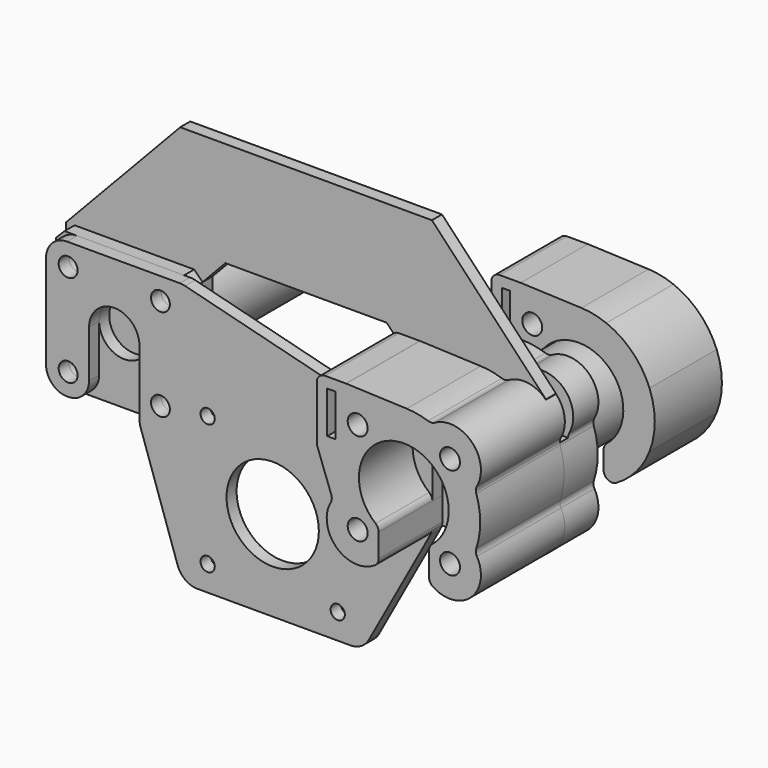
from build123d import *

# Parameters (mm, degrees)
F0_R           = 1.7
F0_R_2         = 11
F0_R_3         = 2.25
F1_DEPTH       = 3
F2_R           = 5
F3_W           = 32.5
F3_H           = 32.5
F3_R           = 2.25
F3_R_2         = 6
F4_DEPTH       = 3
F5_R           = 10.5
F5_R_2         = 6
F6_DEPTH       = 50
F7_SIZE        = 2
F10_R          = 2.375
F10_W          = 2
F10_H          = 10
F11_DEPTH      = 10
F13_R          = 2.375
F13_W          = 2
F13_H          = 10
F14_DEPTH      = 20
F12_W          = 2.5
F12_H          = 12.5
F15_DEPTH      = 36.626
F17_DEPTH      = 3
F18_F1_R       = 2
F18_F2_R       = 2
F18_2_T1_DEPTH = 25.630870957
F18_2_T3_DEPTH = 25.0205555548
F18_2_T5_DEPTH = 27.4736016845
F18_2_T7_DEPTH = 21.7710498822
F18_2_T9_DEPTH = 30
F19_R          = 2.25
F20_DEPTH      = 3
F21_R          = 1.99999
F21_R_2        = 2
F22_R          = 2.375
F23_DEPTH      = 3
F24_R          = 3.5
F26_R          = 2.375
F27_DEPTH      = 25


# Not quite as in the source:
# - a fillet or chamfer that OpenCascade refuses, or shapes differently, is made with other operations: its cross-section is extruded or revolved along the edge and cut away or added
# - a fillet or chamfer is up to 0.001 mm smaller than in the source, because OpenCascade refuses the exact size
# - an extrude whose draft closes it to a point is written as a loft to that point


with BuildPart() as f1:
    # F0 (on Front) → F1 (new body)
    with BuildSketch(Plane.XZ):
        with BuildLine():
            Line((-24.65, 16.25), (-57.15, 16.25))
            Line((-57.15, 16.25), (-57.15, -16.25))
            Line((-57.15, -16.25), (-46.9, -16.25))
            Line((-46.9, -16.25), (-46.9, 0))
            ThreePointArc((-46.9, 0), (-40.9, 6), (-34.9, 0))
            Line((-34.9, 0), (-34.9, -16.25))
            Line((-34.9, -16.25), (-24.65, -46.5))
            Line((-24.65, -46.5), (18.35, -46.5))
            Line((18.35, -46.5), (34.9, -16.25))
            Line((34.9, -16.25), (34.9, 0))
            ThreePointArc((34.9, 0), (40.9, 6), (46.9, 0))
            Line((46.9, 0), (46.9, -16.25))
            Line((46.9, -16.25), (57.15, -16.25))
            Line((57.15, -16.25), (57.15, 16.25))
            Line((57.15, 16.25), (24.65, 16.25))
            Line((24.65, 16.25), (24.65, 6.25))
            Line((24.65, 6.25), (14.65, 6.25))
            Line((14.65, 6.25), (-24.65, 16.25))
        make_face()
        with Locations((-18.65, -40.5)):
            Circle(F0_R, mode=Mode.SUBTRACT)
        with Locations((-3.15, -25)):
            Circle(F0_R_2, mode=Mode.SUBTRACT)
        with Locations((12.35, -40.5)):
            Circle(F0_R, mode=Mode.SUBTRACT)
        with Locations((-51.9, -11)):
            Circle(F0_R_3, mode=Mode.SUBTRACT)
        with Locations((-29.9, -11)):
            Circle(F0_R_3, mode=Mode.SUBTRACT)
        with Locations((-18.65, -9.5)):
            Circle(F0_R, mode=Mode.SUBTRACT)
        with Locations((-51.9, 11)):
            Circle(F0_R_3, mode=Mode.SUBTRACT)
        with Locations((-29.9, 11)):
            Circle(F0_R_3, mode=Mode.SUBTRACT)
        with Locations((12.35, -9.5)):
            Circle(F0_R, mode=Mode.SUBTRACT)
        with Locations((29.9, -11)):
            Circle(F0_R_3, mode=Mode.SUBTRACT)
        with Locations((51.9, -11)):
            Circle(F0_R_3, mode=Mode.SUBTRACT)
        with Locations((29.9, 11)):
            Circle(F0_R_3, mode=Mode.SUBTRACT)
        with Locations((51.9, 11)):
            Circle(F0_R_3, mode=Mode.SUBTRACT)
    extrude(amount=F1_DEPTH)

    # F2
    f2_edges = [f1.edges().sort_by_distance(p)[0] for p in [
        (-57.15, -1.5, -16.25),
        (-57.15, -1.5, 16.25),
        (-46.9, -1.5, -16.25),
        (-34.9, -1.5, -16.25),
        (-24.65, -1.5, -46.5),
        (18.35, -1.5, -46.5),
        (34.9, -1.5, -16.25),
        (46.9, -1.5, -16.25),
        (57.15, -1.5, -16.25),
        (57.15, -1.5, 16.25),
        (24.65, -1.5, 16.25),
        (14.65, -1.5, 6.25),
        (-24.65, -1.5, 16.25),
    ]]
    fillet(f2_edges, radius=F2_R)


with BuildPart() as f4:
    # F3 (on face) → F4 (new body)
    with BuildSketch(Plane(origin=(0, 0, 0), x_dir=(-1, 0, 0), z_dir=(0, 1, 0))):
        with Locations((-40.9, 0)):
            Rectangle(F3_W, F3_H)
        with Locations((-51.9, -11)):
            Circle(F3_R, mode=Mode.SUBTRACT)
        with Locations((-29.9, -11)):
            Circle(F3_R, mode=Mode.SUBTRACT)
        with Locations((-51.9, 11)):
            Circle(F3_R, mode=Mode.SUBTRACT)
        with Locations((-40.9, 0)):
            Circle(F3_R_2, mode=Mode.SUBTRACT)
        with Locations((-29.9, 11)):
            Circle(F3_R, mode=Mode.SUBTRACT)
    extrude(amount=F4_DEPTH)

    # F5 (on face) → F6 (join)
    with BuildSketch(Plane(origin=(0, 3, 0), x_dir=(-1, 0, 0), z_dir=(0, 1, 0))):
        with Locations((-40.9, 0)):
            Circle(F5_R)
        with Locations((-40.9, 0)):
            Circle(F5_R_2, mode=Mode.SUBTRACT)
    extrude(amount=F6_DEPTH)

    # F7
    f7_edges = [f4.edges().sort_by_distance(p)[0] for p in [
        (57.15, 1.5, 16.25),
        (24.65, 1.5, 16.25),
        (24.65, 1.5, -16.25),
        (57.15, 1.5, -16.25),
    ]]
    chamfer(f7_edges, length=F7_SIZE)


with BuildPart() as f8_1:
    # F8: instance of F4
    add(f4.part.mirror(Plane.YZ))


with BuildPart() as f11:
    # F10 (on offset) → F11 (new body)
    with BuildSketch(Plane(origin=(0, 6, 0), x_dir=(-1, 0, 0), z_dir=(0, 1, 0))):
        with BuildLine():
            ThreePointArc((-46.9, -8.8594582227), (-40.9, 10.7), (-34.9, -8.8594582227))
            Line((-34.9, -8.8594582227), (-34.9, -16.4213121106))
            ThreePointArc((-34.9, -16.4213121106), (-24.9853159914, -16.4987731446), (-23.9535532643, -6.6376157643))
            ThreePointArc((-23.9535532643, -6.6376157643), (-23.8791795551, -6.4445070705), (-23.8070062826, -6.2505652365))
            Line((-23.8070062826, -6.2505652365), (-20.15, 3.75))
            Line((-20.15, 3.75), (-20.15, 18.75))
            Line((-20.15, 18.75), (-27.15, 18.75))
            Line((-27.15, 18.75), (-41.609153009, 18.1861788733))
            ThreePointArc((-41.609153009, 18.1861788733), (-44.625317006, 17.8146572576), (-47.5376157643, 16.9464467357))
            ThreePointArc((-47.5376157643, 16.9464467357), (-57.1149125113, 16.2149125113), (-57.8464467357, 6.6376157643))
            ThreePointArc((-57.8464467357, 6.6376157643), (-59.1, 0), (-57.8464467357, -6.6376157643))
            ThreePointArc((-57.8464467357, -6.6376157643), (-56.8146840086, -16.4987731446), (-46.9, -16.4213121106))
            Line((-46.9, -16.4213121106), (-46.9, -8.8594582227))
        make_face()
        with Locations((-51.9, -11)):
            Circle(F10_R, mode=Mode.SUBTRACT)
        with Locations((-29.9, -11)):
            Circle(F10_R, mode=Mode.SUBTRACT)
        with Locations((-51.9, 11)):
            Circle(F10_R, mode=Mode.SUBTRACT)
        with Locations((-29.9, 11)):
            Circle(F10_R, mode=Mode.SUBTRACT)
        with Locations((-23.65, 11.25)):
            Rectangle(F10_W, F10_H, mode=Mode.SUBTRACT)
    extrude(amount=F11_DEPTH)

    # F12 (on face) → F15 (cut, through all)
    with BuildSketch(Plane.YZ.offset(22.65)):
        with Locations((7.25, 12.5)):
            Rectangle(F12_W, F12_H)
    extrude(amount=F15_DEPTH, mode=Mode.SUBTRACT)

    # F16 (on face) → F17 (cut)
    with BuildSketch(Plane(origin=(0, 16, 0), x_dir=(-1, 0, 0), z_dir=(0, 1, 0))):
        Polygon((-47.9962572492, 9.9539952825), (-49.0422619668, 13.8577380332), (-52.9460047175, 14.9037427508), (-55.8037427508, 12.0460047175), (-54.7577380332, 8.1422619668), (-50.8539952825, 7.0962572492), align=None)
        Polygon((-50.8539952825, -7.0962572492), (-54.7577380332, -8.1422619668), (-55.8037427508, -12.0460047175), (-52.9460047175, -14.9037427508), (-49.0422619668, -13.8577380332), (-47.9962572492, -9.9539952825), align=None)
    extrude(amount=-F17_DEPTH, mode=Mode.SUBTRACT)

    # F18: fillet of radius 2 on 11 edges, made by hand

    # F18_f1
    f18_f1_edges = [f11.edges().sort_by_distance(p)[0] for p in [
        (47.5376157643, 12.25, 16.9464467357),
        (57.8464467357, 12.25, 6.6376157643),
        (57.8464467357, 11, -6.6376157643),
        (23.9535532643, 11, -6.6376157643),
    ]]
    fillet(f18_f1_edges, radius=F18_F1_R)

    # F18_f2
    f18_f2_edges = [f11.edges().sort_by_distance(p)[0] for p in [
        (46.9, 11, -16.4213121106),
        (46.9, 11, -8.8594582227),
        (20.15, 11, 3.75),
        (20.15, 11, 18.75),
        (27.15, 12.25, 18.75),
        (34.9, 11, -8.8594582227),
        (34.9, 11, -16.4213121106),
    ]]
    fillet(f18_f2_edges, radius=F18_F2_R)

    # F24 (on face) → F25 section 0
    with BuildSketch(Plane(origin=(0, 16, 0), x_dir=(-1, 0, 0), z_dir=(0, 1, 0)), mode=Mode.PRIVATE) as f25_s0:
        with Locations((-29.9, -11)):
            Circle(F24_R)
    loft([f25_s0.sketch, Vertex(29.9, 12.5, -11)], ruled=True, mode=Mode.SUBTRACT)


with BuildPart() as f14:
    # F13 (on face) → F14 (new body)
    with BuildSketch(Plane(origin=(0, 53, 0), x_dir=(-1, 0, 0), z_dir=(0, 1, 0))):
        with BuildLine():
            Line((-27.15, 18.75), (-41.609153009, 18.1861788733))
            ThreePointArc((-41.609153009, 18.1861788733), (-44.625317006, 17.8146572576), (-47.5376157643, 16.9464467357))
            ThreePointArc((-47.5376157643, 16.9464467357), (-53.7693434176, 12.8693434176), (-57.8464467357, 6.6376157643))
            ThreePointArc((-57.8464467357, 6.6376157643), (-59.1, 0), (-57.8464467357, -6.6376157643))
            ThreePointArc((-57.8464467357, -6.6376157643), (-53.7693434176, -12.8693434176), (-47.5376157643, -16.9464467357))
            ThreePointArc((-47.5376157643, -16.9464467357), (-47.2114499856, -16.6928133434), (-46.9, -16.4213121106))
            Line((-46.9, -16.4213121106), (-46.9, -8.8594582227))
            ThreePointArc((-46.9, -8.8594582227), (-40.9, 10.7), (-34.9, -8.8594582227))
            Line((-34.9, -8.8594582227), (-34.9, -16.4213121106))
            ThreePointArc((-34.9, -16.4213121106), (-34.5885500144, -16.6928133434), (-34.2623842357, -16.9464467357))
            ThreePointArc((-34.2623842357, -16.9464467357), (-28.0306565824, -12.8693434176), (-23.9535532643, -6.6376157643))
            ThreePointArc((-23.9535532643, -6.6376157643), (-23.8791795551, -6.4445070705), (-23.8070062826, -6.2505652365))
            Line((-23.8070062826, -6.2505652365), (-20.15, 3.75))
            Line((-20.15, 3.75), (-20.15, 18.75))
            Line((-20.15, 18.75), (-27.15, 18.75))
        make_face()
        with Locations((-29.9, 11)):
            Circle(F13_R, mode=Mode.SUBTRACT)
        with Locations((-23.65, 11.25)):
            Rectangle(F13_W, F13_H, mode=Mode.SUBTRACT)
    extrude(amount=-F14_DEPTH)

    # F18#2: fillet of radius 2 on 6 edges, made by hand

    # F18_2_s2 → F18_2_t1 (cut)
    with BuildSketch(Plane.XZ.offset(-55.8154354785)):
        with BuildLine():
            ThreePointArc((46.9, -15.4598906937), (47.1347014219, -16.3999550161), (47.7837209302, -17.1193849053))
            ThreePointArc((47.7837209302, -17.1193849053), (47.3285163868, -16.7872413613), (46.9, -16.4213121106))
            Line((46.9, -16.4213121106), (46.9, -15.4598906937))
        make_face()
    extrude(amount=F18_2_T1_DEPTH, mode=Mode.SUBTRACT)

    # F18_2_s4 → F18_2_t3 (cut)
    with BuildSketch(Plane.XZ.offset(-55.5102777774)):
        with BuildLine():
            ThreePointArc((47.6401574803, -8.3102513284), (47.0944966021, -9.0032452783), (46.9, -9.8635693337))
            Line((46.9, -9.8635693337), (46.9, -8.8594582227))
            ThreePointArc((46.9, -8.8594582227), (47.2759948407, -8.5928278111), (47.6401574803, -8.3102513284))
        make_face()
        with BuildLine():
            ThreePointArc((34.9, -9.8635693337), (34.7055033979, -9.0032452783), (34.1598425197, -8.3102513284))
            ThreePointArc((34.1598425197, -8.3102513284), (34.5240051593, -8.5928278111), (34.9, -8.8594582227))
            Line((34.9, -8.8594582227), (34.9, -9.8635693337))
        make_face()
    extrude(amount=F18_2_T3_DEPTH, mode=Mode.SUBTRACT)

    # F18_2_s6 → F18_2_t5 (cut)
    with BuildSketch(Plane.XZ.offset(-56.7368008423)):
        with BuildLine():
            ThreePointArc((35.3717736883, -15.9447262517), (34.2737734044, -16.5662065114), (33.0222118523, -16.4067197788))
            ThreePointArc((33.0222118523, -16.4067197788), (33.6372826037, -16.6881076225), (34.2623842357, -16.9464467357))
            ThreePointArc((34.2623842357, -16.9464467357), (34.8425222812, -16.4737645638), (35.3717736883, -15.9447262517))
        make_face()
    extrude(amount=F18_2_T5_DEPTH, mode=Mode.SUBTRACT)

    # F18_2_s8 → F18_2_t7 (cut)
    with BuildSketch(Plane.XZ.offset(-53.8855249411)):
        with BuildLine():
            ThreePointArc((20.271649042, 3.4173346757), (20.1806470713, 3.7554277492), (20.15, 4.1042099764))
            Line((20.15, 4.1042099764), (20.15, 3.75))
            Line((20.15, 3.75), (20.271649042, 3.4173346757))
        make_face()
    extrude(amount=F18_2_T7_DEPTH, mode=Mode.SUBTRACT)

    # F18_2_s10 → F18_2_t9 (cut)
    with BuildSketch(Plane.XZ.offset(-58)):
        with BuildLine():
            ThreePointArc((22.15, 18.75), (20.7357864376, 18.1642135624), (20.15, 16.75))
            Line((20.15, 16.75), (20.15, 18.75))
            Line((20.15, 18.75), (22.15, 18.75))
        make_face()
    extrude(amount=F18_2_T9_DEPTH, mode=Mode.SUBTRACT)

    # F21#2 (call 1 of 2: OpenCascade refuses the feature's edges together) (radius 2 in the source; OpenCascade refuses exactly that, so slightly less here)
    f21_2_edges = [f14.edges().sort_by_distance(p)[0] for p in [
        (47.554648, 43, -16.939765),
    ]]
    fillet(f21_2_edges, radius=F21_R)

    # F21 (call 2 of 2)
    f21_edges = [f14.edges().sort_by_distance(p)[0] for p in [
        (34.9, 43, -16.328794),
    ]]
    fillet(f21_edges, radius=F21_R_2)

    # F22 (on face) → F23 (cut)
    with BuildSketch(Plane(origin=(0, 53, 0), x_dir=(-1, 0, 0), z_dir=(0, 1, 0))):
        Polygon((-26.4, 13.0207259422), (-29.9, 15.0414518843), (-33.4, 13.0207259422), (-33.4, 8.9792740578), (-29.9, 6.9585481157), (-26.4, 8.9792740578), align=None)
        with Locations((-29.9, 11)):
            Circle(F22_R, mode=Mode.SUBTRACT)
    extrude(amount=-F23_DEPTH, mode=Mode.SUBTRACT)


with BuildPart() as f20:
    # F19 (on face) → F20 (new body)
    with BuildSketch(Plane(origin=(0, 3, 0), x_dir=(-1, 0, 0), z_dir=(0, 1, 0))):
        Polygon((-29.9941596701, 45), (-57.15, 16.25), (-57.15, -16.25), (-24.65, -16.25), (-24.65, 14.25), (-19.218831934, 20), (0, 20), (19.218831934, 20), (24.65, 14.25), (24.65, -16.25), (57.15, -16.25), (57.15, 16.25), (29.9941596701, 45), (0, 45), align=None)
        with Locations((-51.9, -11)):
            Circle(F19_R, mode=Mode.SUBTRACT)
        with Locations((-29.9, -11)):
            Circle(F19_R, mode=Mode.SUBTRACT)
        with Locations((-51.9, 11)):
            Circle(F19_R, mode=Mode.SUBTRACT)
        with Locations((-29.9, 11)):
            Circle(F19_R, mode=Mode.SUBTRACT)
        with Locations((29.9, -11)):
            Circle(F19_R, mode=Mode.SUBTRACT)
        with Locations((51.9, -11)):
            Circle(F19_R, mode=Mode.SUBTRACT)
        with Locations((29.9, 11)):
            Circle(F19_R, mode=Mode.SUBTRACT)
        with Locations((51.9, 11)):
            Circle(F19_R, mode=Mode.SUBTRACT)
    extrude(amount=F20_DEPTH)


with BuildPart() as f27:
    # F26 (on face) → F27 (new body)
    with BuildSketch(Plane.XZ.offset(-6)):
        with BuildLine():
            ThreePointArc((34.0162790698, -17.1193849053), (34.6652985781, -16.3999550161), (34.9, -15.4598906937))
            Line((34.9, -15.4598906937), (34.9, -9.8635693337))
            ThreePointArc((34.9, -9.8635693337), (34.7055033979, -9.0032452783), (34.1598425197, -8.3102513284))
            ThreePointArc((34.1598425197, -8.3102513284), (30.2941839268, -1.4165681848), (32.2150993097, 6.25))
            Line((32.2150993097, 6.25), (24.65, 6.25))
            Line((24.65, 6.25), (22.65, 6.25))
            Line((22.65, 6.25), (22.65, 16.25))
            Line((22.65, 16.25), (22.65, 18.75))
            Line((22.65, 18.75), (22.15, 18.75))
            ThreePointArc((22.15, 18.75), (20.7357864376, 18.1642135624), (20.15, 16.75))
            Line((20.15, 16.75), (20.15, 4.1042099764))
            ThreePointArc((20.15, 4.1042099764), (20.1806470713, 3.7554277492), (20.271649042, 3.4173346757))
            Line((20.271649042, 3.4173346757), (23.6100791686, -5.7120421119))
            ThreePointArc((23.6100791686, -5.7120421119), (23.7251373809, -6.5611514408), (23.4742928591, -7.380481698))
            ThreePointArc((23.4742928591, -7.380481698), (24.8955096738, -16.4171673018), (34.0162790698, -17.1193849053))
        make_face()
        with Locations((29.9, -11)):
            Circle(F26_R, mode=Mode.SUBTRACT)
        with BuildLine():
            Line((24.65, 6.25), (32.2150993097, 6.25))
            ThreePointArc((32.2150993097, 6.25), (40.9, 10.7), (49.5849006903, 6.25))
            Line((49.5849006903, 6.25), (58.0677434676, 6.25))
            ThreePointArc((58.0677434676, 6.25), (58.1120564954, 6.830133642), (58.321467254, 7.3729649429))
            ThreePointArc((58.321467254, 7.3729649429), (57.1149125113, 16.2149125113), (48.2729649429, 17.421467254))
            ThreePointArc((48.2729649429, 17.421467254), (47.4813913058, 17.1721222405), (46.6567520952, 17.2655670429))
            ThreePointArc((46.6567520952, 17.2655670429), (44.1655571867, 17.9046400763), (41.609153009, 18.1861788733))
            Line((41.609153009, 18.1861788733), (27.1889496506, 18.7484811949))
            ThreePointArc((27.1889496506, 18.7484811949), (27.1499925991, 18.7496202627), (27.1110207485, 18.75))
            Line((27.1110207485, 18.75), (22.65, 18.75))
            Line((22.65, 18.75), (22.65, 16.25))
            Line((22.65, 16.25), (24.65, 16.25))
            Line((24.65, 16.25), (24.65, 6.25))
        make_face()
        with Locations((29.9, 11)):
            Circle(F26_R, mode=Mode.SUBTRACT)
        with Locations((51.9, 11)):
            Circle(F26_R, mode=Mode.SUBTRACT)
        with BuildLine():
            Line((58.0677434676, 6.25), (49.5849006903, 6.25))
            ThreePointArc((49.5849006903, 6.25), (51.5058160732, -1.4165681848), (47.6401574803, -8.3102513284))
            ThreePointArc((47.6401574803, -8.3102513284), (47.0944966021, -9.0032452783), (46.9, -9.8635693337))
            Line((46.9, -9.8635693337), (46.9, -15.4598906937))
            ThreePointArc((46.9, -15.4598906937), (47.1347014219, -16.3999550161), (47.7837209302, -17.1193849053))
            ThreePointArc((47.7837209302, -17.1193849053), (56.9076590002, -16.4142382971), (58.321467254, -7.3729649429))
            ThreePointArc((58.321467254, -7.3729649429), (58.0721222405, -6.5813913058), (58.1655670429, -5.7567520952))
            ThreePointArc((58.1655670429, -5.7567520952), (59.1, 0), (58.1655670429, 5.7567520952))
            ThreePointArc((58.1655670429, 5.7567520952), (58.1010915136, 6.0002893627), (58.0677434676, 6.25))
        make_face()
        with Locations((51.9, -11)):
            Circle(F26_R, mode=Mode.SUBTRACT)
    extrude(amount=F27_DEPTH)


solid = Compound([f1.part, f4.part, f8_1.part, f11.part, f14.part, f20.part, f27.part])
